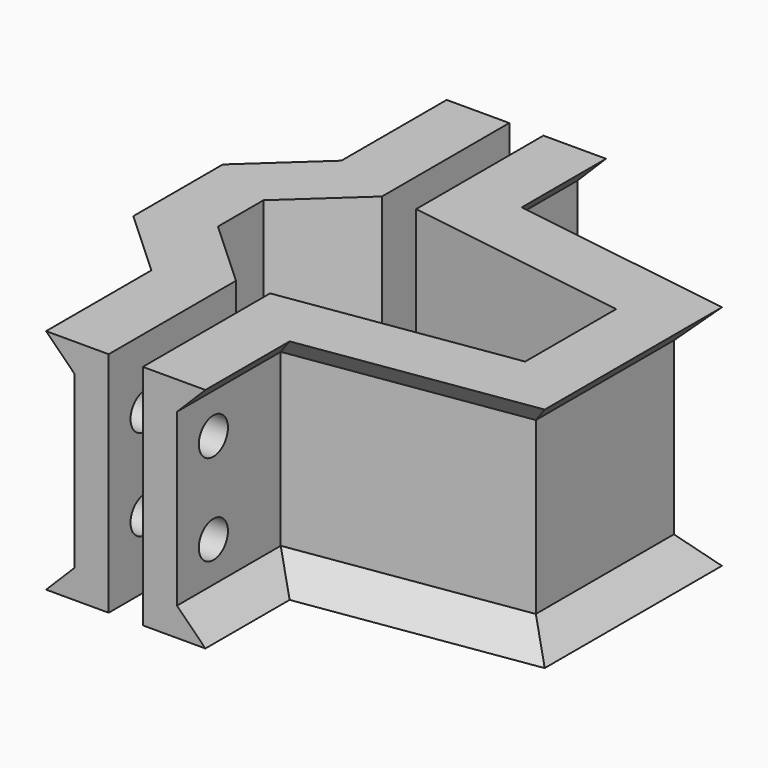
from build123d import *

# Parameters (mm, degrees)
F1_DEPTH   = 10
F2_R       = 1.6
F3_DEPTH   = 3
F5_DEPTH   = 10
F6_R       = 1.6
F7_DEPTH   = 3
F9_DEPTH   = 2.5
F11_DEPTH  = 2.5
F12_SIZE   = 2.49999
F12_2_SIZE = 2.49999


# Not quite as in the source:
# - a fillet or chamfer is up to 0.001 mm smaller than in the source, because OpenCascade refuses the exact size


with BuildPart() as f1:
    # F0 (on Top) → F1 (new body)
    with BuildSketch(Plane.XY):
        Polygon((-3, -22), (0, -22), (0, -8.0198083574), (-6, -2.5), (-6, 2.5), (0, 8.0198083574), (0, 22), (-3, 22), (-3, 9.3363083632), (-9, 3.8165000058), (-9, 0), (-9, -3.8165000058), (-3, -9.3363083632), align=None)
    extrude(amount=F1_DEPTH)

    # F2 (on face) → F3 (cut, through all)
    with BuildSketch(Plane.YZ):
        with Locations((-18, 6)):
            Circle(F2_R)
        with Locations((18, 6)):
            Circle(F2_R)
    extrude(amount=-F3_DEPTH, mode=Mode.SUBTRACT)

    # F8 (on face) → F9 (join)
    with BuildSketch(Plane(origin=(0, 0, 0), x_dir=(1, 0, 0), z_dir=(0, 0, -1))):
        Polygon((-3, 9.3363083632), (-3, 22), (-5.5, 22), (-5.5, 10.4333917014), (-11.5, 4.913583344), (-11.5, -4.913583344), (-5.5, -10.4333917014), (-5.5, -22), (-3, -22), (-3, -9.3363083632), (-9, -3.8165000058), (-9, 3.8165000058), align=None)
    extrude(amount=-F9_DEPTH)

    # F12#2 (size 2.5 in the source; OpenCascade refuses exactly that, so slightly less here)
    f12_2_edges = [f1.edges().sort_by_distance(p)[0] for p in [
        (-5.5, 16.216696, 2.5),
        (-8.5, 7.673488, 2.5),
        (-11.5, 0, 2.5),
        (-8.5, -7.673488, 2.5),
        (-5.5, -16.216696, 2.5),
    ]]
    chamfer(f12_2_edges, length=F12_2_SIZE)



with BuildPart() as f5:
    # F4 (on Top) → F5 (new body)
    with BuildSketch(Plane.XY):
        Polygon((3, -8.0198083574), (3, -22), (6, -22), (6, -10.6008415462), (26, -7.5810331888), (26, 7.5810331888), (6, 10.6008415462), (6, 22), (3, 22), (3, 8.0198083574), (23, 5), (23, 0), (23, -5), align=None)
    extrude(amount=F5_DEPTH)

    # F6 (on face) → F7 (cut, through all)
    with BuildSketch(Plane.YZ.offset(6)):
        with Locations((-18, 6)):
            Circle(F6_R)
        with Locations((18, 6)):
            Circle(F6_R)
    extrude(amount=-F7_DEPTH, mode=Mode.SUBTRACT)

    # F10 (on face) → F11 (join)
    with BuildSketch(Plane(origin=(0, 0, 0), x_dir=(1, 0, 0), z_dir=(0, 0, -1))):
        Polygon((6, -10.6008415462), (6, -22), (8.5, -22), (8.5, -12.7517025368), (28.5, -9.7318941795), (28.5, 9.7318941795), (8.5, 12.7517025368), (8.5, 22), (6, 22), (6, 10.6008415462), (26, 7.5810331888), (26, -7.5810331888), align=None)
    extrude(amount=-F11_DEPTH)

    # F12 (size 2.5 in the source; OpenCascade refuses exactly that, so slightly less here)
    f12_edges = [f5.edges().sort_by_distance(p)[0] for p in [
        (8.5, 17.375851, 2.5),
        (18.5, 11.241798, 2.5),
        (28.5, 0, 2.5),
        (18.5, -11.241798, 2.5),
        (8.5, -17.375851, 2.5),
    ]]
    chamfer(f12_edges, length=F12_SIZE)


with BuildPart() as f1_1:
    add(f1.part)

    add(f5.part)  # F13 merges F5
    # F13: F1, F5 across face
    add(f1.part.mirror(Plane(origin=(-3.2621858931, 0, 10), x_dir=(1, 0, 0), z_dir=(0, 0, 1))))
    add(f5.part.mirror(Plane(origin=(-3.2621858931, 0, 10), x_dir=(1, 0, 0), z_dir=(0, 0, 1))))


solid = f1_1.part
